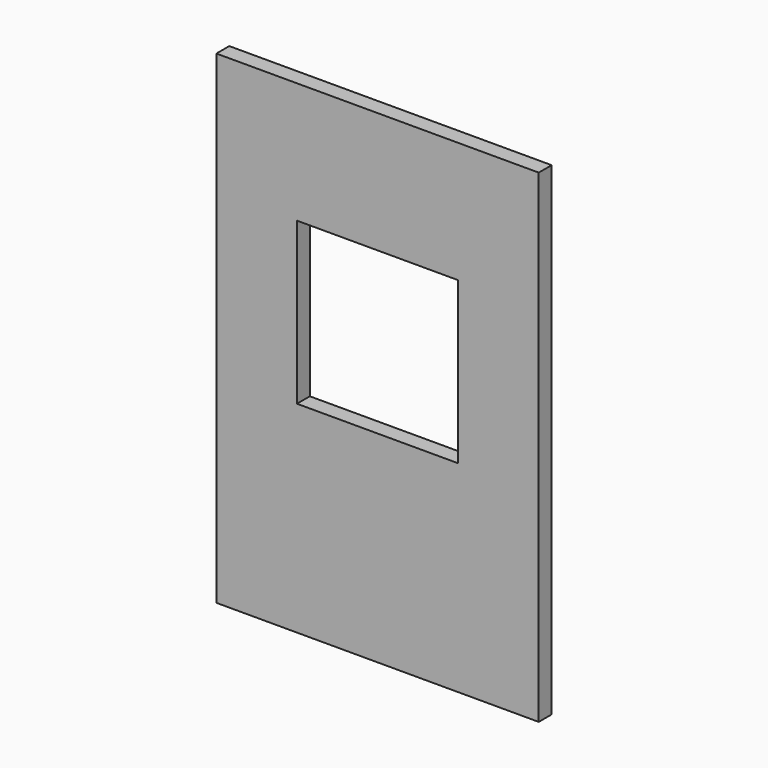
from build123d import *

# Parameters (mm, degrees)
F0_W     = 2000
F0_H     = 3000
F1_DEPTH = 50
F2_W     = 1000
F2_H     = 1000
F3_DEPTH = 100.001


# Not quite as in the source:
# - a feature names something its author has since deleted; it is built from what else it names


with BuildPart() as f1:
    # F0 (on Front) → F1 (new body, symmetric)
    with BuildSketch(Plane.XZ):
        with Locations((0, 1500)):
            Rectangle(F0_W, F0_H)
    extrude(amount=F1_DEPTH, both=True)

    # F2 (on face) → F3 (cut, through all)
    with BuildSketch(Plane.XZ.offset(50)):
        with Locations((0, 1750)):
            Rectangle(F2_W, F2_H)
    extrude(amount=-F3_DEPTH, mode=Mode.SUBTRACT)


solid = f1.part
